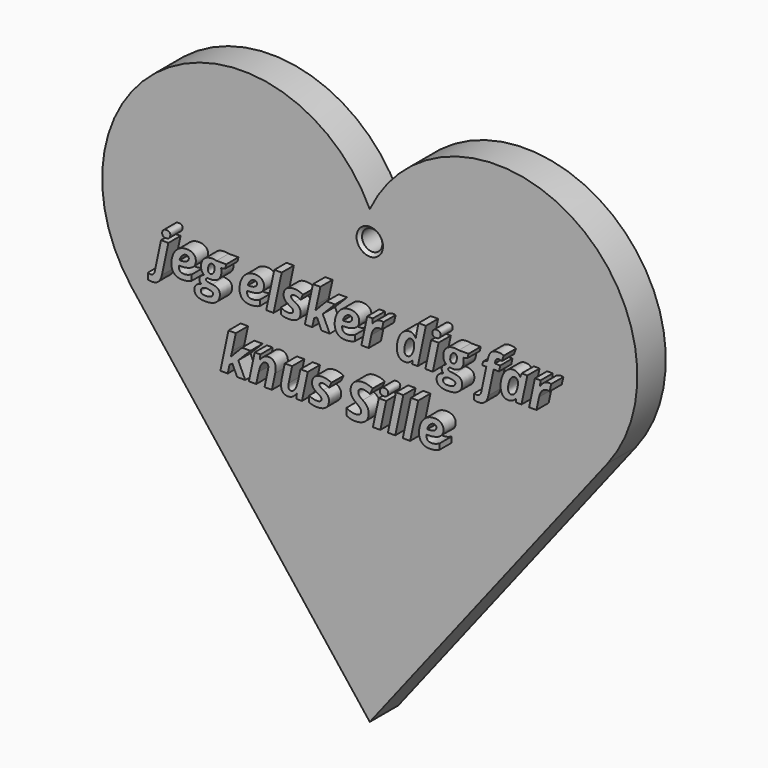
from build123d import *

# Parameters (mm, degrees)
F1_DEPTH       = 7
F2_TEXT_SIZE   = 9.8776864606
F4_DEPTH       = 3
F6_D           = 4
F6_DEPTH       = 60
F6_CSINK_D     = 5.2
F6_CSINK_ANGLE = 90
F6_TIP         = 1.2017212381


# Not quite as in the source:
# - Text() gives the source's letters only with a copy of the font that has no kerning and outlines rounded to 1/6400 em; it was checked with that copy


with BuildPart() as f1:
    # F0 (on Front) → F1 (new body)
    with BuildSketch(Plane.XZ):
        with BuildLine():
            ThreePointArc((46.7965012793, 0), (39.4855968326, 40.5426199141), (0, 28.7935350094))
            ThreePointArc((0, 28.7935350094), (-39.4855968326, 40.5426199141), (-46.7965012793, 0))
            Line((-46.7965012793, 0), (0, -60))
            Line((0, -60), (46.7965012793, 0))
        make_face()
    extrude(amount=F1_DEPTH)

    # F2 (on face) → F4 (join)
    with BuildSketch(Plane.XZ.offset(7)):
        with Locations((-40, 6.6816007577)):
            Text('jeg elsker dig far', F2_TEXT_SIZE, font='Open Sans', font_style=FontStyle.BOLDITALIC, text_align=(TextAlign.LEFT, TextAlign.BOTTOM))
        with Locations((-27.1667245437, -6.7520528287)):
            Text('knus Sille', F2_TEXT_SIZE, font='Open Sans', font_style=FontStyle.BOLDITALIC, text_align=(TextAlign.LEFT, TextAlign.BOTTOM))
    extrude(amount=F4_DEPTH)

    # F6
    with Locations(Plane.XZ.offset(7)):
        with Locations((0, 23.1760870665)):
            CounterSinkHole(F6_D / 2, F6_CSINK_D / 2, depth=F6_DEPTH, counter_sink_angle=F6_CSINK_ANGLE)
            with Locations((0, 0, -(F6_DEPTH + F6_TIP / 2))):  # 118° drill point
                Cone(0, F6_D / 2, F6_TIP, mode=Mode.SUBTRACT)


solid = f1.part
